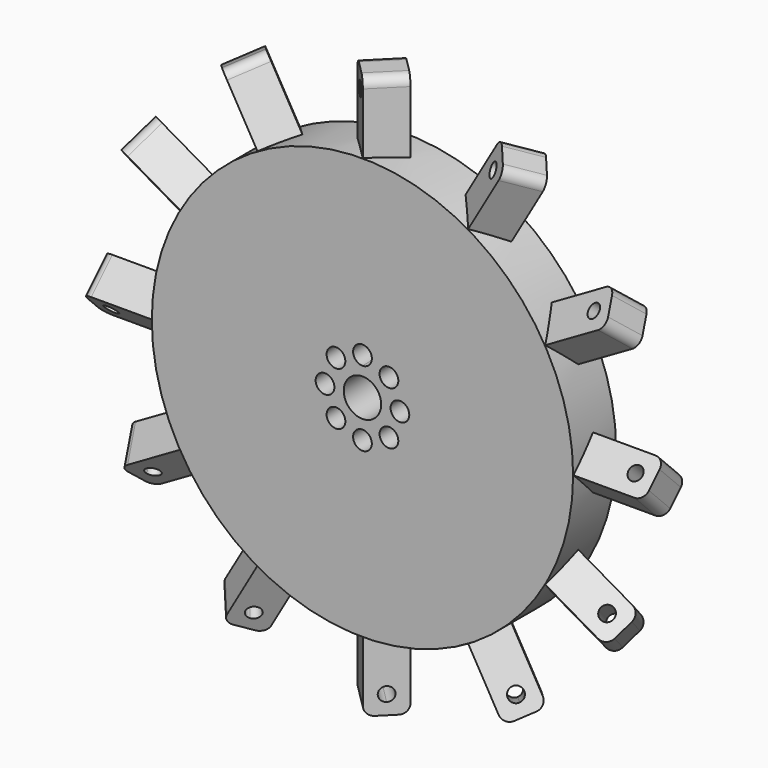
from build123d import *

# Parameters (mm, degrees)
F2_W            = 4
F2_H            = 60
F3_DEPTH        = 4
F3_COPIES_COUNT = 12
F4_R            = 45
F5_DEPTH        = 5.75
F7_DEPTH        = 25
F7_COPIES_COUNT = 12
F8_R            = 2
F9_R            = 2
F10_DEPTH       = 25


# Not quite as in the source:
# - a pattern or mirror of a feature is missing from the dataset's text; its kind, count and spacing are read off the source's solid


with BuildPart() as f3:
    # F2 (on face) → F3 (new body, symmetric)
    with BuildSketch(Plane(origin=(0, 0, 0), x_dir=(-0.7071067812, 0.7071067812, 0), z_dir=(0.7071067812, 0.7071067812, 0))):
        with Locations((-2, 30)):
            Rectangle(F2_W, F2_H)
        with Locations((2, 30)):
            Rectangle(F2_W, F2_H)
    extrude(amount=F3_DEPTH, both=True)

    # F3_copies: F3 ×12 about axis
    f3_copies_axis = Axis((0, 0, 0), (0, 1, 0))


with BuildPart() as f3_1:
    add(f3.part)
    for i in range(1, F3_COPIES_COUNT):
        add(f3.part.rotate(f3_copies_axis, i * 360 / F3_COPIES_COUNT))

    # F4 (on Front) → F5 (join, symmetric)
    with BuildSketch(Plane.XZ):
        Circle(F4_R)
    extrude(amount=F5_DEPTH, both=True)

    # F6 (on face) → F7 (cut)
    with BuildSketch(Plane(origin=(-2.8284271247, -2.8284271247, 0), x_dir=(0.7071067812, -0.7071067812, 0), z_dir=(-0.7071067812, -0.7071067812, 0))):
        with BuildLine():
            ThreePointArc((1.5, 56), (1.0606601718, 57.0606601718), (0, 57.5))
            ThreePointArc((0, 57.5), (-1.0606601718, 54.9393398282), (1.5, 56))
        make_face()
    f7 = extrude(amount=-F7_DEPTH, mode=Mode.SUBTRACT)

    # F7_copies: F7 ×12 about axis
    f7_copies_axis = Axis((0, 0, 0), (0, 1, 0))
    for i in range(1, F7_COPIES_COUNT):
        add(f7.rotate(f7_copies_axis, i * 360 / F7_COPIES_COUNT), mode=Mode.SUBTRACT)

    # F8
    f8_edges = [f3_1.edges().sort_by_distance(p)[0] for p in [
        (2.828427, -2.828427, 60),
        (-2.828427, 2.828427, 60),
        (60, 2.828427, 2.828427),
        (60, -2.828427, -2.828427),
        (53.375738, -2.828427, 27.55051),
        (50.547311, 2.828427, 32.44949),
        (32.44949, -2.828427, 50.547311),
        (27.55051, 2.828427, 53.375738),
        (-32.44949, 2.828427, 50.547311),
        (-27.55051, -2.828427, 53.375738),
        (-53.375738, 2.828427, 27.55051),
        (-50.547311, -2.828427, 32.44949),
        (-60, 2.828427, -2.828427),
        (-60, -2.828427, 2.828427),
        (-50.547311, 2.828427, -32.44949),
        (-53.375738, -2.828427, -27.55051),
        (-27.55051, 2.828427, -53.375738),
        (-32.44949, -2.828427, -50.547311),
        (27.55051, -2.828427, -53.375738),
        (32.44949, 2.828427, -50.547311),
        (50.547311, -2.828427, -32.44949),
        (53.375738, 2.828427, -27.55051),
        (2.828427, 2.828427, -60),
        (-2.828427, -2.828427, -60),
    ]]
    fillet(f8_edges, radius=F8_R)

    # F9 (on face) → F10 (cut)
    with BuildSketch(Plane.XZ.offset(5.75)):
        with BuildLine():
            ThreePointArc((0, 4), (-2.8284271247, -2.8284271247), (4, 0))
            ThreePointArc((4, 0), (2.8284271247, 2.8284271247), (0, 4))
        make_face()
        with BuildLine():
            ThreePointArc((2, 8), (-1.4142135624, 9.4142135624), (0, 6))
            ThreePointArc((0, 6), (1.4142135624, 6.5857864376), (2, 8))
        make_face()
        with Locations((-5.6568542495, 5.6568542495)):
            Circle(F9_R)
        with Locations((-8, 0)):
            Circle(F9_R)
        with Locations((-5.6568542495, -5.6568542495)):
            Circle(F9_R)
        with Locations((0, -8)):
            Circle(F9_R)
        with Locations((5.6568542495, -5.6568542495)):
            Circle(F9_R)
        with Locations((8, 0)):
            Circle(F9_R)
        with Locations((5.6568542495, 5.6568542495)):
            Circle(F9_R)
    extrude(amount=-F10_DEPTH, mode=Mode.SUBTRACT)


solid = f3_1.part
